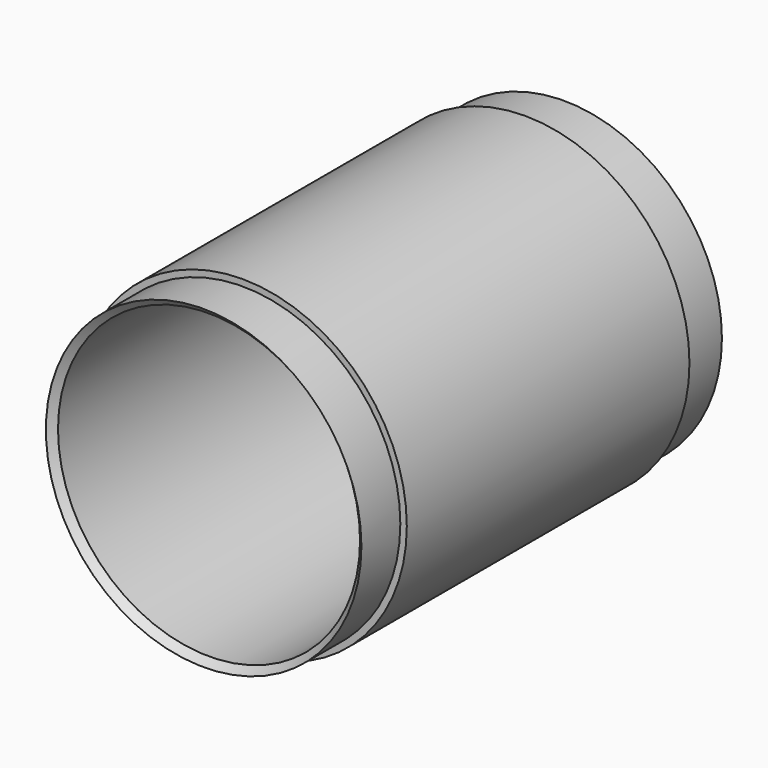
from build123d import *

# Parameters (mm, degrees)
F0_R     = 63.5
F0_R_2   = 58.39
F1_DEPTH = 175
F2_R     = 63.5
F2_R_2   = 61
F3_DEPTH = 19.2
F4_R     = 63.5
F4_R_2   = 61
F5_DEPTH = 19.2


# Not quite as in the source:
# - a fillet or chamfer that OpenCascade refuses, or shapes differently, is made with other operations: its cross-section is extruded or revolved along the edge and cut away or added


with BuildPart() as f1:
    # F0 (on Front) → F1 (new body)
    with BuildSketch(Plane.XZ):
        Circle(F0_R)
        Circle(F0_R_2, mode=Mode.SUBTRACT)
    extrude(amount=F1_DEPTH)

    # F2 (on Front) → F3 (cut)
    with BuildSketch(Plane.XZ):
        Circle(F2_R)
        Circle(F2_R_2, mode=Mode.SUBTRACT)
    extrude(amount=F3_DEPTH, mode=Mode.SUBTRACT)

    # F4 (on face) → F5 (cut)
    with BuildSketch(Plane.XZ.offset(175)):
        Circle(F4_R)
        Circle(F4_R_2, mode=Mode.SUBTRACT)
    extrude(amount=-F5_DEPTH, mode=Mode.SUBTRACT)

    # F6: chamfer of 3 on 2 edges, made by hand

    # F6_s1 → F6_t2 (revolve, cut)
    with BuildSketch(Plane.XY):
        Polygon((61.39, -175), (58.39, -172), (58.39, -175), align=None)
    revolve(axis=Axis((0, -175, 0), (0, -1, 0)), mode=Mode.SUBTRACT)

    # F6_s3 → F6_t4 (revolve, cut)
    with BuildSketch(Plane.XY):
        Polygon((61.39, 0), (58.39, -3), (58.39, 0), align=None)
    revolve(axis=Axis((0, 0, 0), (0, -1, 0)), mode=Mode.SUBTRACT)


solid = f1.part
